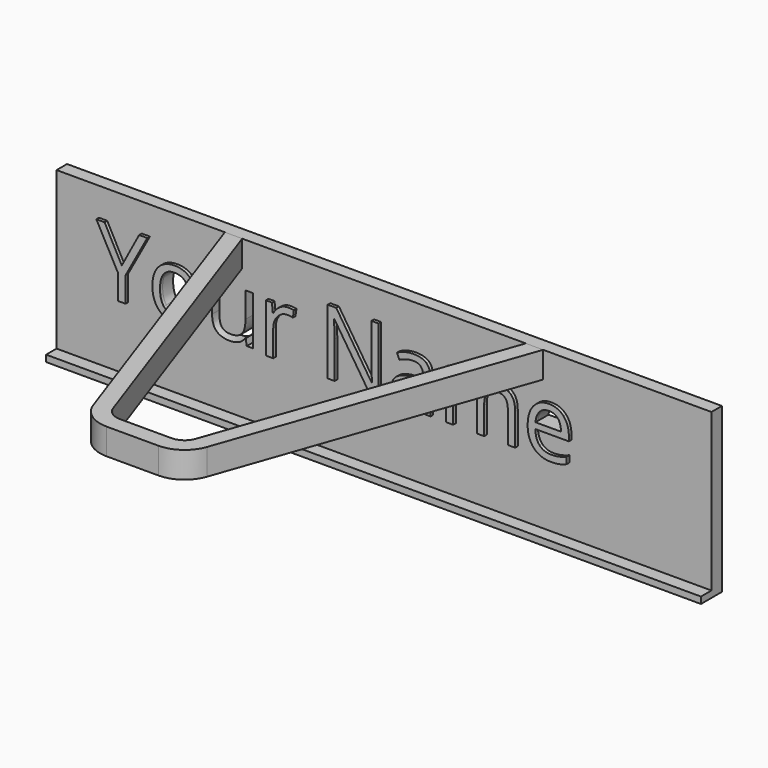
from build123d import *

# Parameters (mm, degrees)
F0_W     = 100
F0_H     = 22
F0_H_2   = 2
F1_DEPTH = 2
F0_H_3   = 1
F2_DEPTH = 4
F4_DEPTH = 4
F5_DEPTH = 2.5


# Not quite as in the source:
# - a feature names something its author has since deleted; it is built from what else it names


with BuildPart() as f1:
    # F0 (on Front) → F1 (new body)
    with BuildSketch(Plane.XZ):
        with Locations((-50, 12)):
            Rectangle(F0_W, F0_H)
        with BuildLine():
            add(Edge.make_bspline(
                [(-79.0596093072, 17.3149081237), (-78.1405554877, 16.2764966653), (-78.1405554877, 14.5078334709)],
                knots=[0, 0, 0, 1, 1, 1], degree=2))
            add(Edge.make_bspline(
                [(-78.1405554877, 14.5078334709), (-78.1405554877, 12.689257082), (-79.0552690294, 11.6682067348)],
                knots=[0, 0, 0, 1, 1, 1], degree=2))
            add(Edge.make_bspline(
                [(-79.0552690294, 11.6682067348), (-79.9699825711, 10.6471563876), (-81.5845659044, 10.6471563876)],
                knots=[0, 0, 0, 1, 1, 1], degree=2))
            add(Edge.make_bspline(
                [(-81.5845659044, 10.6471563876), (-82.5828297933, 10.6471563876), (-83.3553992377, 11.1159063876)],
                knots=[0, 0, 0, 1, 1, 1], degree=2))
            add(Edge.make_bspline(
                [(-83.3553992377, 11.1159063876), (-84.1279686822, 11.5846563876), (-84.5489756266, 12.4592223598)],
                knots=[0, 0, 0, 1, 1, 1], degree=2))
            add(Edge.make_bspline(
                [(-84.5489756266, 12.4592223598), (-84.9699825711, 13.333788332), (-84.9699825711, 14.5078334709)],
                knots=[0, 0, 0, 1, 1, 1], degree=2))
            add(Edge.make_bspline(
                [(-84.9699825711, 14.5078334709), (-84.9699825711, 16.3242397209), (-84.0606943766, 17.3387796515)],
                knots=[0, 0, 0, 1, 1, 1], degree=2))
            add(Edge.make_bspline(
                [(-84.0606943766, 17.3387796515), (-83.1514061822, 18.353319582), (-81.5368228488, 18.353319582)],
                knots=[0, 0, 0, 1, 1, 1], degree=2))
            add(Edge.make_bspline(
                [(-81.5368228488, 18.353319582), (-79.9786631266, 18.353319582), (-79.0596093072, 17.3149081237)],
                knots=[0, 0, 0, 1, 1, 1], degree=2))
        make_face(mode=Mode.SUBTRACT)
        Polygon((-92.2659895155, 20.6992397209), (-89.64012146, 15.7404723598), (-86.9968922933, 20.6992397209), (-85.7490624322, 20.6992397209), (-89.0585242377, 14.6293612487), (-89.0585242377, 10.7838751376), (-90.2238888211, 10.7838751376), (-90.2238888211, 14.5751077765), (-93.52684021, 20.6992397209), align=None, mode=Mode.SUBTRACT)
        with BuildLine():
            Line((-76.2460242377, 18.216600832), (-75.1067013211, 18.216600832))
            Line((-75.1067013211, 18.216600832), (-75.1067013211, 13.3945522209))
            add(Edge.make_bspline(
                [(-75.1067013211, 13.3945522209), (-75.1067013211, 12.4852640265), (-74.6932898627, 12.0382154153)],
                knots=[0, 0, 0, 1, 1, 1], degree=2))
            add(Edge.make_bspline(
                [(-74.6932898627, 12.0382154153), (-74.2798784044, 11.5911668042), (-73.3988020155, 11.5911668042)],
                knots=[0, 0, 0, 1, 1, 1], degree=2))
            add(Edge.make_bspline(
                [(-73.3988020155, 11.5911668042), (-72.2312672933, 11.5911668042), (-71.6930728488, 12.2281025681)],
                knots=[0, 0, 0, 1, 1, 1], degree=2))
            add(Edge.make_bspline(
                [(-71.6930728488, 12.2281025681), (-71.1548784044, 12.865038332), (-71.1548784044, 14.310350832)],
                knots=[0, 0, 0, 1, 1, 1], degree=2))
            Line((-71.1548784044, 14.310350832), (-71.1548784044, 18.216600832))
            Line((-71.1548784044, 18.216600832), (-70.0285763211, 18.216600832))
            Line((-70.0285763211, 18.216600832), (-70.0285763211, 10.7838751376))
            Line((-70.0285763211, 10.7838751376), (-70.9573957655, 10.7838751376))
            Line((-70.9573957655, 10.7838751376), (-71.1201561822, 11.7799688876))
            Line((-71.1201561822, 11.7799688876), (-71.1809200711, 11.7799688876))
            add(Edge.make_bspline(
                [(-71.1809200711, 11.7799688876), (-71.5259721544, 11.2309237487), (-72.14012146, 10.9390400681)],
                knots=[0, 0, 0, 1, 1, 1], degree=2))
            add(Edge.make_bspline(
                [(-72.14012146, 10.9390400681), (-72.7542707655, 10.6471563876), (-73.5420311822, 10.6471563876)],
                knots=[0, 0, 0, 1, 1, 1], degree=2))
            add(Edge.make_bspline(
                [(-73.5420311822, 10.6471563876), (-74.8983679877, 10.6471563876), (-75.5721961127, 11.2916876376)],
                knots=[0, 0, 0, 1, 1, 1], degree=2))
            add(Edge.make_bspline(
                [(-75.5721961127, 11.2916876376), (-76.2460242377, 11.9362188876), (-76.2460242377, 13.353319582)],
                knots=[0, 0, 0, 1, 1, 1], degree=2))
            Line((-76.2460242377, 13.353319582), (-76.2460242377, 18.216600832))
        make_face(mode=Mode.SUBTRACT)
        with BuildLine():
            add(Edge.make_bspline(
                [(-65.5320485433, 17.9594393737), (-64.9482811822, 18.353319582), (-64.24949646, 18.353319582)],
                knots=[0, 0, 0, 1, 1, 1], degree=2))
            add(Edge.make_bspline(
                [(-64.24949646, 18.353319582), (-63.7547047933, 18.353319582), (-63.3619096544, 18.2708543042)],
                knots=[0, 0, 0, 1, 1, 1], degree=2))
            Line((-63.3619096544, 18.2708543042), (-63.5181596544, 17.2270174987))
            add(Edge.make_bspline(
                [(-63.5181596544, 17.2270174987), (-63.9782290988, 17.3290140265), (-64.3319617377, 17.3290140265)],
                knots=[0, 0, 0, 1, 1, 1], degree=2))
            add(Edge.make_bspline(
                [(-64.3319617377, 17.3290140265), (-65.2347395155, 17.3290140265), (-65.8749304877, 16.5965921515)],
                knots=[0, 0, 0, 1, 1, 1], degree=2))
            add(Edge.make_bspline(
                [(-65.8749304877, 16.5965921515), (-66.51512146, 15.8641702765), (-66.51512146, 14.7725904153)],
                knots=[0, 0, 0, 1, 1, 1], degree=2))
            Line((-66.51512146, 14.7725904153), (-66.51512146, 10.7838751376))
            Line((-66.51512146, 10.7838751376), (-67.6414235433, 10.7838751376))
            Line((-67.6414235433, 10.7838751376), (-67.6414235433, 18.216600832))
            Line((-67.6414235433, 18.216600832), (-66.7126040988, 18.216600832))
            Line((-66.7126040988, 18.216600832), (-66.5823957655, 16.8407327765))
            Line((-66.5823957655, 16.8407327765), (-66.5281422933, 16.8407327765))
            add(Edge.make_bspline(
                [(-66.5281422933, 16.8407327765), (-66.1158159044, 17.5655591653), (-65.5320485433, 17.9594393737)],
                knots=[0, 0, 0, 1, 1, 1], degree=2))
        make_face(mode=Mode.SUBTRACT)
        with BuildLine():
            Line((-50.4474131266, 20.6992397209), (-50.4474131266, 10.7838751376))
            Line((-50.4474131266, 10.7838751376), (-51.7625172933, 10.7838751376))
            Line((-51.7625172933, 10.7838751376), (-57.1813540988, 19.1041876376))
            Line((-57.1813540988, 19.1041876376), (-57.2356075711, 19.1041876376))
            add(Edge.make_bspline(
                [(-57.2356075711, 19.1041876376), (-57.1271006266, 17.6393438876), (-57.1271006266, 16.419725832)],
                knots=[0, 0, 0, 1, 1, 1], degree=2))
            Line((-57.1271006266, 16.419725832), (-57.1271006266, 10.7838751376))
            Line((-57.1271006266, 10.7838751376), (-58.1926388211, 10.7838751376))
            Line((-58.1926388211, 10.7838751376), (-58.1926388211, 20.6992397209))
            Line((-58.1926388211, 20.6992397209), (-56.8905554877, 20.6992397209))
            Line((-56.8905554877, 20.6992397209), (-51.4847395155, 12.4114793042))
            Line((-51.4847395155, 12.4114793042), (-51.4304860433, 12.4114793042))
            add(Edge.make_bspline(
                [(-51.4304860433, 12.4114793042), (-51.4435068766, 12.5937709709), (-51.4912499322, 13.587694582)],
                knots=[0, 0, 0, 1, 1, 1], degree=2))
            add(Edge.make_bspline(
                [(-51.4912499322, 13.587694582), (-51.5389929877, 14.5816181931), (-51.5259721544, 15.0091355542)],
                knots=[0, 0, 0, 1, 1, 1], degree=2))
            Line((-51.5259721544, 15.0091355542), (-51.5259721544, 20.6992397209))
            Line((-51.5259721544, 20.6992397209), (-50.4474131266, 20.6992397209))
        make_face(mode=Mode.SUBTRACT)
        with BuildLine():
            Line((-42.4851735433, 10.7838751376), (-43.3206770155, 10.7838751376))
            Line((-43.3206770155, 10.7838751376), (-43.5442013211, 11.8429029153))
            Line((-43.5442013211, 11.8429029153), (-43.5984547933, 11.8429029153))
            add(Edge.make_bspline(
                [(-43.5984547933, 11.8429029153), (-44.1540103488, 11.1441181931), (-44.7063106961, 10.8956372903)],
                knots=[0, 0, 0, 1, 1, 1], degree=2))
            add(Edge.make_bspline(
                [(-44.7063106961, 10.8956372903), (-45.2586110433, 10.6471563876), (-46.0876040988, 10.6471563876)],
                knots=[0, 0, 0, 1, 1, 1], degree=2))
            add(Edge.make_bspline(
                [(-46.0876040988, 10.6471563876), (-47.1922047933, 10.6471563876), (-47.8193749322, 11.2179029153)],
                knots=[0, 0, 0, 1, 1, 1], degree=2))
            add(Edge.make_bspline(
                [(-47.8193749322, 11.2179029153), (-48.4465450711, 11.7886494431), (-48.4465450711, 12.8389966653)],
                knots=[0, 0, 0, 1, 1, 1], degree=2))
            add(Edge.make_bspline(
                [(-48.4465450711, 12.8389966653), (-48.4465450711, 15.0894306931), (-44.8462846544, 15.1979376376)],
                knots=[0, 0, 0, 1, 1, 1], degree=2))
            Line((-44.8462846544, 15.1979376376), (-43.58543396, 15.2391702765))
            Line((-43.58543396, 15.2391702765), (-43.58543396, 15.7014098598))
            add(Edge.make_bspline(
                [(-43.58543396, 15.7014098598), (-43.58543396, 16.575975832), (-43.9608679877, 16.9926424987)],
                knots=[0, 0, 0, 1, 1, 1], degree=2))
            add(Edge.make_bspline(
                [(-43.9608679877, 16.9926424987), (-44.3363020155, 17.4093091653), (-45.1652950711, 17.4093091653)],
                knots=[0, 0, 0, 1, 1, 1], degree=2))
            add(Edge.make_bspline(
                [(-45.1652950711, 17.4093091653), (-46.0941145155, 17.4093091653), (-47.2659895155, 16.8407327765)],
                knots=[0, 0, 0, 1, 1, 1], degree=2))
            Line((-47.2659895155, 16.8407327765), (-47.6132117377, 17.7022779153))
            add(Edge.make_bspline(
                [(-47.6132117377, 17.7022779153), (-47.0641665988, 17.9995869431), (-46.4098697238, 18.1688577765)],
                knots=[0, 0, 0, 1, 1, 1], degree=2))
            add(Edge.make_bspline(
                [(-46.4098697238, 18.1688577765), (-45.7555728488, 18.3381286098), (-45.0958506266, 18.3381286098)],
                knots=[0, 0, 0, 1, 1, 1], degree=2))
            add(Edge.make_bspline(
                [(-45.0958506266, 18.3381286098), (-43.7677256266, 18.3381286098), (-43.126449585, 17.7489359015)],
                knots=[0, 0, 0, 1, 1, 1], degree=2))
            add(Edge.make_bspline(
                [(-43.126449585, 17.7489359015), (-42.4851735433, 17.1597431931), (-42.4851735433, 15.8576598598)],
                knots=[0, 0, 0, 1, 1, 1], degree=2))
            Line((-42.4851735433, 15.8576598598), (-42.4851735433, 10.7838751376))
        make_face(mode=Mode.SUBTRACT)
        with BuildLine():
            Line((-29.5685068766, 10.7838751376), (-30.6926388211, 10.7838751376))
            Line((-30.6926388211, 10.7838751376), (-30.6926388211, 15.618944582))
            add(Edge.make_bspline(
                [(-30.6926388211, 15.618944582), (-30.6926388211, 16.5087015265), (-31.0724131266, 16.9524949292)],
                knots=[0, 0, 0, 1, 1, 1], degree=2))
            add(Edge.make_bspline(
                [(-31.0724131266, 16.9524949292), (-31.4521874322, 17.396288332), (-32.2529686822, 17.396288332)],
                knots=[0, 0, 0, 1, 1, 1], degree=2))
            add(Edge.make_bspline(
                [(-32.2529686822, 17.396288332), (-33.3033159044, 17.396288332), (-33.8057030572, 16.7929897209)],
                knots=[0, 0, 0, 1, 1, 1], degree=2))
            add(Edge.make_bspline(
                [(-33.8057030572, 16.7929897209), (-34.30809021, 16.1896911098), (-34.30809021, 14.935350832)],
                knots=[0, 0, 0, 1, 1, 1], degree=2))
            Line((-34.30809021, 14.935350832), (-34.30809021, 10.7838751376))
            Line((-34.30809021, 10.7838751376), (-35.4343922933, 10.7838751376))
            Line((-35.4343922933, 10.7838751376), (-35.4343922933, 15.618944582))
            add(Edge.make_bspline(
                [(-35.4343922933, 15.618944582), (-35.4343922933, 16.5087015265), (-35.8141665988, 16.9524949292)],
                knots=[0, 0, 0, 1, 1, 1], degree=2))
            add(Edge.make_bspline(
                [(-35.8141665988, 16.9524949292), (-36.1939409044, 17.396288332), (-37.0012325711, 17.396288332)],
                knots=[0, 0, 0, 1, 1, 1], degree=2))
            add(Edge.make_bspline(
                [(-37.0012325711, 17.396288332), (-38.05809021, 17.396288332), (-38.5496266683, 16.7626077765)],
                knots=[0, 0, 0, 1, 1, 1], degree=2))
            add(Edge.make_bspline(
                [(-38.5496266683, 16.7626077765), (-39.0411631266, 16.1289272209), (-39.0411631266, 14.6836147209)],
                knots=[0, 0, 0, 1, 1, 1], degree=2))
            Line((-39.0411631266, 14.6836147209), (-39.0411631266, 10.7838751376))
            Line((-39.0411631266, 10.7838751376), (-40.16746521, 10.7838751376))
            Line((-40.16746521, 10.7838751376), (-40.16746521, 18.216600832))
            Line((-40.16746521, 18.216600832), (-39.2516665988, 18.216600832))
            Line((-39.2516665988, 18.216600832), (-39.0693749322, 17.1988056931))
            Line((-39.0693749322, 17.1988056931), (-39.01512146, 17.1988056931))
            add(Edge.make_bspline(
                [(-39.01512146, 17.1988056931), (-38.6961110433, 17.7413404153), (-38.1155988905, 18.0473299987)],
                knots=[0, 0, 0, 1, 1, 1], degree=2))
            add(Edge.make_bspline(
                [(-38.1155988905, 18.0473299987), (-37.5350867377, 18.353319582), (-36.8167707655, 18.353319582)],
                knots=[0, 0, 0, 1, 1, 1], degree=2))
            add(Edge.make_bspline(
                [(-36.8167707655, 18.353319582), (-35.0741492377, 18.353319582), (-34.5381249322, 17.0902987487)],
                knots=[0, 0, 0, 1, 1, 1], degree=2))
            Line((-34.5381249322, 17.0902987487), (-34.48387146, 17.0902987487))
            add(Edge.make_bspline(
                [(-34.48387146, 17.0902987487), (-34.15184021, 17.6740661098), (-33.5214148627, 18.0136928459)],
                knots=[0, 0, 0, 1, 1, 1], degree=2))
            add(Edge.make_bspline(
                [(-33.5214148627, 18.0136928459), (-32.8909895155, 18.353319582), (-32.0836978488, 18.353319582)],
                knots=[0, 0, 0, 1, 1, 1], degree=2))
            add(Edge.make_bspline(
                [(-32.0836978488, 18.353319582), (-30.8228471544, 18.353319582), (-30.1956770155, 17.7055331237)],
                knots=[0, 0, 0, 1, 1, 1], degree=2))
            add(Edge.make_bspline(
                [(-30.1956770155, 17.7055331237), (-29.5685068766, 17.0577466653), (-29.5685068766, 15.6319654153)],
                knots=[0, 0, 0, 1, 1, 1], degree=2))
            Line((-29.5685068766, 15.6319654153), (-29.5685068766, 10.7838751376))
        make_face(mode=Mode.SUBTRACT)
        with BuildLine():
            add(Edge.make_bspline(
                [(-22.82371521, 10.7600036098), (-23.3553992377, 10.6471563876), (-24.1084374322, 10.6471563876)],
                knots=[0, 0, 0, 1, 1, 1], degree=2))
            add(Edge.make_bspline(
                [(-24.1084374322, 10.6471563876), (-25.7555728488, 10.6471563876), (-26.7093488905, 11.6519306931)],
                knots=[0, 0, 0, 1, 1, 1], degree=2))
            add(Edge.make_bspline(
                [(-26.7093488905, 11.6519306931), (-27.6631249322, 12.6567049987), (-27.6631249322, 14.4383890265)],
                knots=[0, 0, 0, 1, 1, 1], degree=2))
            add(Edge.make_bspline(
                [(-27.6631249322, 14.4383890265), (-27.6631249322, 16.2374341653), (-26.7777082655, 17.2953768737)],
                knots=[0, 0, 0, 1, 1, 1], degree=2))
            add(Edge.make_bspline(
                [(-26.7777082655, 17.2953768737), (-25.8922915988, 18.353319582), (-24.3992360433, 18.353319582)],
                knots=[0, 0, 0, 1, 1, 1], degree=2))
            add(Edge.make_bspline(
                [(-24.3992360433, 18.353319582), (-23.0038367377, 18.353319582), (-22.1900346544, 17.4342657626)],
                knots=[0, 0, 0, 1, 1, 1], degree=2))
            add(Edge.make_bspline(
                [(-22.1900346544, 17.4342657626), (-21.3762325711, 16.5152119431), (-21.3762325711, 15.0091355542)],
                knots=[0, 0, 0, 1, 1, 1], degree=2))
            Line((-21.3762325711, 15.0091355542), (-21.3762325711, 14.2973299987))
            Line((-21.3762325711, 14.2973299987), (-26.49559021, 14.2973299987))
            add(Edge.make_bspline(
                [(-26.49559021, 14.2973299987), (-26.4608679877, 12.9887362487), (-25.8336978488, 12.3105678459)],
                knots=[0, 0, 0, 1, 1, 1], degree=2))
            add(Edge.make_bspline(
                [(-25.8336978488, 12.3105678459), (-25.20652771, 11.6323994431), (-24.0672047933, 11.6323994431)],
                knots=[0, 0, 0, 1, 1, 1], degree=2))
            add(Edge.make_bspline(
                [(-24.0672047933, 11.6323994431), (-22.8671179877, 11.6323994431), (-21.6952429877, 12.1337015265)],
                knots=[0, 0, 0, 1, 1, 1], degree=2))
            Line((-21.6952429877, 12.1337015265), (-21.6952429877, 11.1289272209))
            add(Edge.make_bspline(
                [(-21.6952429877, 11.1289272209), (-22.2920311822, 10.872850832), (-22.82371521, 10.7600036098)],
                knots=[0, 0, 0, 1, 1, 1], degree=2))
        make_face(mode=Mode.SUBTRACT)
        with Locations((-50, 24)):
            Rectangle(F0_W, F0_H_2)
        with BuildLine():
            add(Edge.make_bspline(
                [(-78.1405554877, 14.5078334709), (-78.1405554877, 12.689257082), (-79.0552690294, 11.6682067348)],
                knots=[0, 0, 0, 1, 1, 1], degree=2))
            add(Edge.make_bspline(
                [(-79.0596093072, 17.3149081237), (-78.1405554877, 16.2764966653), (-78.1405554877, 14.5078334709)],
                knots=[0, 0, 0, 1, 1, 1], degree=2))
            add(Edge.make_bspline(
                [(-81.5368228488, 18.353319582), (-79.9786631266, 18.353319582), (-79.0596093072, 17.3149081237)],
                knots=[0, 0, 0, 1, 1, 1], degree=2))
            add(Edge.make_bspline(
                [(-84.0606943766, 17.3387796515), (-83.1514061822, 18.353319582), (-81.5368228488, 18.353319582)],
                knots=[0, 0, 0, 1, 1, 1], degree=2))
            add(Edge.make_bspline(
                [(-84.9699825711, 14.5078334709), (-84.9699825711, 16.3242397209), (-84.0606943766, 17.3387796515)],
                knots=[0, 0, 0, 1, 1, 1], degree=2))
            add(Edge.make_bspline(
                [(-84.5489756266, 12.4592223598), (-84.9699825711, 13.333788332), (-84.9699825711, 14.5078334709)],
                knots=[0, 0, 0, 1, 1, 1], degree=2))
            add(Edge.make_bspline(
                [(-83.3553992377, 11.1159063876), (-84.1279686822, 11.5846563876), (-84.5489756266, 12.4592223598)],
                knots=[0, 0, 0, 1, 1, 1], degree=2))
            add(Edge.make_bspline(
                [(-81.5845659044, 10.6471563876), (-82.5828297933, 10.6471563876), (-83.3553992377, 11.1159063876)],
                knots=[0, 0, 0, 1, 1, 1], degree=2))
            add(Edge.make_bspline(
                [(-79.0552690294, 11.6682067348), (-79.9699825711, 10.6471563876), (-81.5845659044, 10.6471563876)],
                knots=[0, 0, 0, 1, 1, 1], degree=2))
        make_face()
        with BuildLine():
            add(Edge.make_bspline(
                [(-83.8024478488, 14.5078334709), (-83.8024478488, 13.0820522209), (-83.2327863905, 12.3366095126)],
                knots=[0, 0, 0, 1, 1, 1], degree=2))
            add(Edge.make_bspline(
                [(-83.2392968072, 16.6703768737), (-83.8024478488, 15.9444654153), (-83.8024478488, 14.5078334709)],
                knots=[0, 0, 0, 1, 1, 1], degree=2))
            add(Edge.make_bspline(
                [(-81.5715450711, 17.396288332), (-82.6761457655, 17.396288332), (-83.2392968072, 16.6703768737)],
                knots=[0, 0, 0, 1, 1, 1], degree=2))
            add(Edge.make_bspline(
                [(-79.8788367377, 16.6606112487), (-80.4517534044, 17.396288332), (-81.5715450711, 17.396288332)],
                knots=[0, 0, 0, 1, 1, 1], degree=2))
            add(Edge.make_bspline(
                [(-79.3059200711, 14.5078334709), (-79.3059200711, 15.9249341653), (-79.8788367377, 16.6606112487)],
                knots=[0, 0, 0, 1, 1, 1], degree=2))
            add(Edge.make_bspline(
                [(-79.8788367377, 12.3333543042), (-79.3059200711, 13.0755418042), (-79.3059200711, 14.5078334709)],
                knots=[0, 0, 0, 1, 1, 1], degree=2))
            add(Edge.make_bspline(
                [(-81.5585242377, 11.5911668042), (-80.4517534044, 11.5911668042), (-79.8788367377, 12.3333543042)],
                knots=[0, 0, 0, 1, 1, 1], degree=2))
            add(Edge.make_bspline(
                [(-83.2327863905, 12.3366095126), (-82.6631249322, 11.5911668042), (-81.5585242377, 11.5911668042)],
                knots=[0, 0, 0, 1, 1, 1], degree=2))
        make_face(mode=Mode.SUBTRACT)
        with BuildLine():
            Line((-51.7625172933, 10.7838751376), (-50.4474131266, 10.7838751376))
            Line((-50.4474131266, 10.7838751376), (-50.4474131266, 20.6992397209))
            Line((-50.4474131266, 20.6992397209), (-51.5259721544, 20.6992397209))
            Line((-51.5259721544, 20.6992397209), (-51.5259721544, 15.0091355542))
            add(Edge.make_bspline(
                [(-51.4912499322, 13.587694582), (-51.5389929877, 14.5816181931), (-51.5259721544, 15.0091355542)],
                knots=[0, 0, 0, 1, 1, 1], degree=2))
            add(Edge.make_bspline(
                [(-51.4304860433, 12.4114793042), (-51.4435068766, 12.5937709709), (-51.4912499322, 13.587694582)],
                knots=[0, 0, 0, 1, 1, 1], degree=2))
            Line((-51.4304860433, 12.4114793042), (-51.4847395155, 12.4114793042))
            Line((-51.4847395155, 12.4114793042), (-56.8905554877, 20.6992397209))
            Line((-56.8905554877, 20.6992397209), (-58.1926388211, 20.6992397209))
            Line((-58.1926388211, 20.6992397209), (-58.1926388211, 10.7838751376))
            Line((-58.1926388211, 10.7838751376), (-57.1271006266, 10.7838751376))
            Line((-57.1271006266, 10.7838751376), (-57.1271006266, 16.419725832))
            add(Edge.make_bspline(
                [(-57.2356075711, 19.1041876376), (-57.1271006266, 17.6393438876), (-57.1271006266, 16.419725832)],
                knots=[0, 0, 0, 1, 1, 1], degree=2))
            Line((-57.2356075711, 19.1041876376), (-57.1813540988, 19.1041876376))
            Line((-57.1813540988, 19.1041876376), (-51.7625172933, 10.7838751376))
        make_face()
        with BuildLine():
            Line((-30.6926388211, 15.618944582), (-30.6926388211, 10.7838751376))
            Line((-30.6926388211, 10.7838751376), (-29.5685068766, 10.7838751376))
            Line((-29.5685068766, 10.7838751376), (-29.5685068766, 15.6319654153))
            add(Edge.make_bspline(
                [(-30.1956770155, 17.7055331237), (-29.5685068766, 17.0577466653), (-29.5685068766, 15.6319654153)],
                knots=[0, 0, 0, 1, 1, 1], degree=2))
            add(Edge.make_bspline(
                [(-32.0836978488, 18.353319582), (-30.8228471544, 18.353319582), (-30.1956770155, 17.7055331237)],
                knots=[0, 0, 0, 1, 1, 1], degree=2))
            add(Edge.make_bspline(
                [(-33.5214148627, 18.0136928459), (-32.8909895155, 18.353319582), (-32.0836978488, 18.353319582)],
                knots=[0, 0, 0, 1, 1, 1], degree=2))
            add(Edge.make_bspline(
                [(-34.48387146, 17.0902987487), (-34.15184021, 17.6740661098), (-33.5214148627, 18.0136928459)],
                knots=[0, 0, 0, 1, 1, 1], degree=2))
            Line((-34.48387146, 17.0902987487), (-34.5381249322, 17.0902987487))
            add(Edge.make_bspline(
                [(-36.8167707655, 18.353319582), (-35.0741492377, 18.353319582), (-34.5381249322, 17.0902987487)],
                knots=[0, 0, 0, 1, 1, 1], degree=2))
            add(Edge.make_bspline(
                [(-38.1155988905, 18.0473299987), (-37.5350867377, 18.353319582), (-36.8167707655, 18.353319582)],
                knots=[0, 0, 0, 1, 1, 1], degree=2))
            add(Edge.make_bspline(
                [(-39.01512146, 17.1988056931), (-38.6961110433, 17.7413404153), (-38.1155988905, 18.0473299987)],
                knots=[0, 0, 0, 1, 1, 1], degree=2))
            Line((-39.01512146, 17.1988056931), (-39.0693749322, 17.1988056931))
            Line((-39.0693749322, 17.1988056931), (-39.2516665988, 18.216600832))
            Line((-39.2516665988, 18.216600832), (-40.16746521, 18.216600832))
            Line((-40.16746521, 18.216600832), (-40.16746521, 10.7838751376))
            Line((-40.16746521, 10.7838751376), (-39.0411631266, 10.7838751376))
            Line((-39.0411631266, 10.7838751376), (-39.0411631266, 14.6836147209))
            add(Edge.make_bspline(
                [(-38.5496266683, 16.7626077765), (-39.0411631266, 16.1289272209), (-39.0411631266, 14.6836147209)],
                knots=[0, 0, 0, 1, 1, 1], degree=2))
            add(Edge.make_bspline(
                [(-37.0012325711, 17.396288332), (-38.05809021, 17.396288332), (-38.5496266683, 16.7626077765)],
                knots=[0, 0, 0, 1, 1, 1], degree=2))
            add(Edge.make_bspline(
                [(-35.8141665988, 16.9524949292), (-36.1939409044, 17.396288332), (-37.0012325711, 17.396288332)],
                knots=[0, 0, 0, 1, 1, 1], degree=2))
            add(Edge.make_bspline(
                [(-35.4343922933, 15.618944582), (-35.4343922933, 16.5087015265), (-35.8141665988, 16.9524949292)],
                knots=[0, 0, 0, 1, 1, 1], degree=2))
            Line((-35.4343922933, 15.618944582), (-35.4343922933, 10.7838751376))
            Line((-35.4343922933, 10.7838751376), (-34.30809021, 10.7838751376))
            Line((-34.30809021, 10.7838751376), (-34.30809021, 14.935350832))
            add(Edge.make_bspline(
                [(-33.8057030572, 16.7929897209), (-34.30809021, 16.1896911098), (-34.30809021, 14.935350832)],
                knots=[0, 0, 0, 1, 1, 1], degree=2))
            add(Edge.make_bspline(
                [(-32.2529686822, 17.396288332), (-33.3033159044, 17.396288332), (-33.8057030572, 16.7929897209)],
                knots=[0, 0, 0, 1, 1, 1], degree=2))
            add(Edge.make_bspline(
                [(-31.0724131266, 16.9524949292), (-31.4521874322, 17.396288332), (-32.2529686822, 17.396288332)],
                knots=[0, 0, 0, 1, 1, 1], degree=2))
            add(Edge.make_bspline(
                [(-30.6926388211, 15.618944582), (-30.6926388211, 16.5087015265), (-31.0724131266, 16.9524949292)],
                knots=[0, 0, 0, 1, 1, 1], degree=2))
        make_face()
        with BuildLine():
            Line((-43.5442013211, 11.8429029153), (-43.3206770155, 10.7838751376))
            Line((-43.3206770155, 10.7838751376), (-42.4851735433, 10.7838751376))
            Line((-42.4851735433, 10.7838751376), (-42.4851735433, 15.8576598598))
            add(Edge.make_bspline(
                [(-43.126449585, 17.7489359015), (-42.4851735433, 17.1597431931), (-42.4851735433, 15.8576598598)],
                knots=[0, 0, 0, 1, 1, 1], degree=2))
            add(Edge.make_bspline(
                [(-45.0958506266, 18.3381286098), (-43.7677256266, 18.3381286098), (-43.126449585, 17.7489359015)],
                knots=[0, 0, 0, 1, 1, 1], degree=2))
            add(Edge.make_bspline(
                [(-46.4098697238, 18.1688577765), (-45.7555728488, 18.3381286098), (-45.0958506266, 18.3381286098)],
                knots=[0, 0, 0, 1, 1, 1], degree=2))
            add(Edge.make_bspline(
                [(-47.6132117377, 17.7022779153), (-47.0641665988, 17.9995869431), (-46.4098697238, 18.1688577765)],
                knots=[0, 0, 0, 1, 1, 1], degree=2))
            Line((-47.6132117377, 17.7022779153), (-47.2659895155, 16.8407327765))
            add(Edge.make_bspline(
                [(-45.1652950711, 17.4093091653), (-46.0941145155, 17.4093091653), (-47.2659895155, 16.8407327765)],
                knots=[0, 0, 0, 1, 1, 1], degree=2))
            add(Edge.make_bspline(
                [(-43.9608679877, 16.9926424987), (-44.3363020155, 17.4093091653), (-45.1652950711, 17.4093091653)],
                knots=[0, 0, 0, 1, 1, 1], degree=2))
            add(Edge.make_bspline(
                [(-43.58543396, 15.7014098598), (-43.58543396, 16.575975832), (-43.9608679877, 16.9926424987)],
                knots=[0, 0, 0, 1, 1, 1], degree=2))
            Line((-43.58543396, 15.7014098598), (-43.58543396, 15.2391702765))
            Line((-43.58543396, 15.2391702765), (-44.8462846544, 15.1979376376))
            add(Edge.make_bspline(
                [(-48.4465450711, 12.8389966653), (-48.4465450711, 15.0894306931), (-44.8462846544, 15.1979376376)],
                knots=[0, 0, 0, 1, 1, 1], degree=2))
            add(Edge.make_bspline(
                [(-47.8193749322, 11.2179029153), (-48.4465450711, 11.7886494431), (-48.4465450711, 12.8389966653)],
                knots=[0, 0, 0, 1, 1, 1], degree=2))
            add(Edge.make_bspline(
                [(-46.0876040988, 10.6471563876), (-47.1922047933, 10.6471563876), (-47.8193749322, 11.2179029153)],
                knots=[0, 0, 0, 1, 1, 1], degree=2))
            add(Edge.make_bspline(
                [(-44.7063106961, 10.8956372903), (-45.2586110433, 10.6471563876), (-46.0876040988, 10.6471563876)],
                knots=[0, 0, 0, 1, 1, 1], degree=2))
            add(Edge.make_bspline(
                [(-43.5984547933, 11.8429029153), (-44.1540103488, 11.1441181931), (-44.7063106961, 10.8956372903)],
                knots=[0, 0, 0, 1, 1, 1], degree=2))
            Line((-43.5984547933, 11.8429029153), (-43.5442013211, 11.8429029153))
        make_face()
        with BuildLine():
            add(Edge.make_bspline(
                [(-45.8640797933, 11.5781459709), (-44.8115624322, 11.5781459709), (-44.2115190294, 12.1543178459)],
                knots=[0, 0, 0, 1, 1, 1], degree=2))
            add(Edge.make_bspline(
                [(-46.8970659044, 11.8960713181), (-46.5281422933, 11.5781459709), (-45.8640797933, 11.5781459709)],
                knots=[0, 0, 0, 1, 1, 1], degree=2))
            add(Edge.make_bspline(
                [(-47.2659895155, 12.825975832), (-47.2659895155, 12.2139966653), (-46.8970659044, 11.8960713181)],
                knots=[0, 0, 0, 1, 1, 1], degree=2))
            add(Edge.make_bspline(
                [(-46.6735415988, 13.9750643737), (-47.2659895155, 13.6050556931), (-47.2659895155, 12.825975832)],
                knots=[0, 0, 0, 1, 1, 1], degree=2))
            add(Edge.make_bspline(
                [(-44.73777771, 14.3928161098), (-46.0810936822, 14.3450730542), (-46.6735415988, 13.9750643737)],
                knots=[0, 0, 0, 1, 1, 1], degree=2))
            Line((-44.73777771, 14.3928161098), (-43.6114756266, 14.4383890265))
            Line((-43.6114756266, 14.4383890265), (-43.6114756266, 13.7678161098))
            add(Edge.make_bspline(
                [(-44.2115190294, 12.1543178459), (-43.6114756266, 12.7304897209), (-43.6114756266, 13.7678161098)],
                knots=[0, 0, 0, 1, 1, 1], degree=2))
        make_face(mode=Mode.SUBTRACT)
        with BuildLine():
            add(Edge.make_bspline(
                [(-24.1084374322, 10.6471563876), (-25.7555728488, 10.6471563876), (-26.7093488905, 11.6519306931)],
                knots=[0, 0, 0, 1, 1, 1], degree=2))
            add(Edge.make_bspline(
                [(-22.82371521, 10.7600036098), (-23.3553992377, 10.6471563876), (-24.1084374322, 10.6471563876)],
                knots=[0, 0, 0, 1, 1, 1], degree=2))
            add(Edge.make_bspline(
                [(-21.6952429877, 11.1289272209), (-22.2920311822, 10.872850832), (-22.82371521, 10.7600036098)],
                knots=[0, 0, 0, 1, 1, 1], degree=2))
            Line((-21.6952429877, 11.1289272209), (-21.6952429877, 12.1337015265))
            add(Edge.make_bspline(
                [(-24.0672047933, 11.6323994431), (-22.8671179877, 11.6323994431), (-21.6952429877, 12.1337015265)],
                knots=[0, 0, 0, 1, 1, 1], degree=2))
            add(Edge.make_bspline(
                [(-25.8336978488, 12.3105678459), (-25.20652771, 11.6323994431), (-24.0672047933, 11.6323994431)],
                knots=[0, 0, 0, 1, 1, 1], degree=2))
            add(Edge.make_bspline(
                [(-26.49559021, 14.2973299987), (-26.4608679877, 12.9887362487), (-25.8336978488, 12.3105678459)],
                knots=[0, 0, 0, 1, 1, 1], degree=2))
            Line((-26.49559021, 14.2973299987), (-21.3762325711, 14.2973299987))
            Line((-21.3762325711, 14.2973299987), (-21.3762325711, 15.0091355542))
            add(Edge.make_bspline(
                [(-22.1900346544, 17.4342657626), (-21.3762325711, 16.5152119431), (-21.3762325711, 15.0091355542)],
                knots=[0, 0, 0, 1, 1, 1], degree=2))
            add(Edge.make_bspline(
                [(-24.3992360433, 18.353319582), (-23.0038367377, 18.353319582), (-22.1900346544, 17.4342657626)],
                knots=[0, 0, 0, 1, 1, 1], degree=2))
            add(Edge.make_bspline(
                [(-26.7777082655, 17.2953768737), (-25.8922915988, 18.353319582), (-24.3992360433, 18.353319582)],
                knots=[0, 0, 0, 1, 1, 1], degree=2))
            add(Edge.make_bspline(
                [(-27.6631249322, 14.4383890265), (-27.6631249322, 16.2374341653), (-26.7777082655, 17.2953768737)],
                knots=[0, 0, 0, 1, 1, 1], degree=2))
            add(Edge.make_bspline(
                [(-26.7093488905, 11.6519306931), (-27.6631249322, 12.6567049987), (-27.6631249322, 14.4383890265)],
                knots=[0, 0, 0, 1, 1, 1], degree=2))
        make_face()
        with BuildLine():
            add(Edge.make_bspline(
                [(-24.4144270155, 17.4093091653), (-25.3085242377, 17.4093091653), (-25.841293335, 16.8266268737)],
                knots=[0, 0, 0, 1, 1, 1], degree=2))
            add(Edge.make_bspline(
                [(-23.0570051405, 16.8429029153), (-23.5311804877, 17.4093091653), (-24.4144270155, 17.4093091653)],
                knots=[0, 0, 0, 1, 1, 1], degree=2))
            add(Edge.make_bspline(
                [(-22.5828297933, 15.2131286098), (-22.5828297933, 16.2764966653), (-23.0570051405, 16.8429029153)],
                knots=[0, 0, 0, 1, 1, 1], degree=2))
            Line((-22.5828297933, 15.2131286098), (-26.4695485433, 15.2131286098))
            add(Edge.make_bspline(
                [(-25.841293335, 16.8266268737), (-26.3740624322, 16.243944582), (-26.4695485433, 15.2131286098)],
                knots=[0, 0, 0, 1, 1, 1], degree=2))
        make_face(mode=Mode.SUBTRACT)
        Polygon((-86.9968922933, 20.6992397209), (-89.64012146, 15.7404723598), (-92.2659895155, 20.6992397209), (-93.52684021, 20.6992397209), (-90.2238888211, 14.5751077765), (-90.2238888211, 10.7838751376), (-89.0585242377, 10.7838751376), (-89.0585242377, 14.6293612487), (-85.7490624322, 20.6992397209), align=None)
        with BuildLine():
            add(Edge.make_bspline(
                [(-64.24949646, 18.353319582), (-63.7547047933, 18.353319582), (-63.3619096544, 18.2708543042)],
                knots=[0, 0, 0, 1, 1, 1], degree=2))
            add(Edge.make_bspline(
                [(-65.5320485433, 17.9594393737), (-64.9482811822, 18.353319582), (-64.24949646, 18.353319582)],
                knots=[0, 0, 0, 1, 1, 1], degree=2))
            add(Edge.make_bspline(
                [(-66.5281422933, 16.8407327765), (-66.1158159044, 17.5655591653), (-65.5320485433, 17.9594393737)],
                knots=[0, 0, 0, 1, 1, 1], degree=2))
            Line((-66.5281422933, 16.8407327765), (-66.5823957655, 16.8407327765))
            Line((-66.5823957655, 16.8407327765), (-66.7126040988, 18.216600832))
            Line((-66.7126040988, 18.216600832), (-67.6414235433, 18.216600832))
            Line((-67.6414235433, 18.216600832), (-67.6414235433, 10.7838751376))
            Line((-67.6414235433, 10.7838751376), (-66.51512146, 10.7838751376))
            Line((-66.51512146, 10.7838751376), (-66.51512146, 14.7725904153))
            add(Edge.make_bspline(
                [(-65.8749304877, 16.5965921515), (-66.51512146, 15.8641702765), (-66.51512146, 14.7725904153)],
                knots=[0, 0, 0, 1, 1, 1], degree=2))
            add(Edge.make_bspline(
                [(-64.3319617377, 17.3290140265), (-65.2347395155, 17.3290140265), (-65.8749304877, 16.5965921515)],
                knots=[0, 0, 0, 1, 1, 1], degree=2))
            add(Edge.make_bspline(
                [(-63.5181596544, 17.2270174987), (-63.9782290988, 17.3290140265), (-64.3319617377, 17.3290140265)],
                knots=[0, 0, 0, 1, 1, 1], degree=2))
            Line((-63.5181596544, 17.2270174987), (-63.3619096544, 18.2708543042))
        make_face()
    extrude(amount=F1_DEPTH)

    # F0 (on Front) → F2 (join)
    with BuildSketch(Plane.XZ):
        with Locations((-50, 0.5)):
            Rectangle(F0_W, F0_H_3)
    extrude(amount=F2_DEPTH)

    # F0 (on Front) → F5 (join)
    with BuildSketch(Plane.XZ):
        Polygon((-86.9968922933, 20.6992397209), (-89.64012146, 15.7404723598), (-92.2659895155, 20.6992397209), (-93.52684021, 20.6992397209), (-90.2238888211, 14.5751077765), (-90.2238888211, 10.7838751376), (-89.0585242377, 10.7838751376), (-89.0585242377, 14.6293612487), (-85.7490624322, 20.6992397209), align=None)
        with BuildLine():
            add(Edge.make_bspline(
                [(-78.1405554877, 14.5078334709), (-78.1405554877, 12.689257082), (-79.0552690294, 11.6682067348)],
                knots=[0, 0, 0, 1, 1, 1], degree=2))
            add(Edge.make_bspline(
                [(-79.0596093072, 17.3149081237), (-78.1405554877, 16.2764966653), (-78.1405554877, 14.5078334709)],
                knots=[0, 0, 0, 1, 1, 1], degree=2))
            add(Edge.make_bspline(
                [(-81.5368228488, 18.353319582), (-79.9786631266, 18.353319582), (-79.0596093072, 17.3149081237)],
                knots=[0, 0, 0, 1, 1, 1], degree=2))
            add(Edge.make_bspline(
                [(-84.0606943766, 17.3387796515), (-83.1514061822, 18.353319582), (-81.5368228488, 18.353319582)],
                knots=[0, 0, 0, 1, 1, 1], degree=2))
            add(Edge.make_bspline(
                [(-84.9699825711, 14.5078334709), (-84.9699825711, 16.3242397209), (-84.0606943766, 17.3387796515)],
                knots=[0, 0, 0, 1, 1, 1], degree=2))
            add(Edge.make_bspline(
                [(-84.5489756266, 12.4592223598), (-84.9699825711, 13.333788332), (-84.9699825711, 14.5078334709)],
                knots=[0, 0, 0, 1, 1, 1], degree=2))
            add(Edge.make_bspline(
                [(-83.3553992377, 11.1159063876), (-84.1279686822, 11.5846563876), (-84.5489756266, 12.4592223598)],
                knots=[0, 0, 0, 1, 1, 1], degree=2))
            add(Edge.make_bspline(
                [(-81.5845659044, 10.6471563876), (-82.5828297933, 10.6471563876), (-83.3553992377, 11.1159063876)],
                knots=[0, 0, 0, 1, 1, 1], degree=2))
            add(Edge.make_bspline(
                [(-79.0552690294, 11.6682067348), (-79.9699825711, 10.6471563876), (-81.5845659044, 10.6471563876)],
                knots=[0, 0, 0, 1, 1, 1], degree=2))
        make_face()
        with BuildLine():
            add(Edge.make_bspline(
                [(-83.8024478488, 14.5078334709), (-83.8024478488, 13.0820522209), (-83.2327863905, 12.3366095126)],
                knots=[0, 0, 0, 1, 1, 1], degree=2))
            add(Edge.make_bspline(
                [(-83.2392968072, 16.6703768737), (-83.8024478488, 15.9444654153), (-83.8024478488, 14.5078334709)],
                knots=[0, 0, 0, 1, 1, 1], degree=2))
            add(Edge.make_bspline(
                [(-81.5715450711, 17.396288332), (-82.6761457655, 17.396288332), (-83.2392968072, 16.6703768737)],
                knots=[0, 0, 0, 1, 1, 1], degree=2))
            add(Edge.make_bspline(
                [(-79.8788367377, 16.6606112487), (-80.4517534044, 17.396288332), (-81.5715450711, 17.396288332)],
                knots=[0, 0, 0, 1, 1, 1], degree=2))
            add(Edge.make_bspline(
                [(-79.3059200711, 14.5078334709), (-79.3059200711, 15.9249341653), (-79.8788367377, 16.6606112487)],
                knots=[0, 0, 0, 1, 1, 1], degree=2))
            add(Edge.make_bspline(
                [(-79.8788367377, 12.3333543042), (-79.3059200711, 13.0755418042), (-79.3059200711, 14.5078334709)],
                knots=[0, 0, 0, 1, 1, 1], degree=2))
            add(Edge.make_bspline(
                [(-81.5585242377, 11.5911668042), (-80.4517534044, 11.5911668042), (-79.8788367377, 12.3333543042)],
                knots=[0, 0, 0, 1, 1, 1], degree=2))
            add(Edge.make_bspline(
                [(-83.2327863905, 12.3366095126), (-82.6631249322, 11.5911668042), (-81.5585242377, 11.5911668042)],
                knots=[0, 0, 0, 1, 1, 1], degree=2))
        make_face(mode=Mode.SUBTRACT)
        with BuildLine():
            add(Edge.make_bspline(
                [(-64.24949646, 18.353319582), (-63.7547047933, 18.353319582), (-63.3619096544, 18.2708543042)],
                knots=[0, 0, 0, 1, 1, 1], degree=2))
            add(Edge.make_bspline(
                [(-65.5320485433, 17.9594393737), (-64.9482811822, 18.353319582), (-64.24949646, 18.353319582)],
                knots=[0, 0, 0, 1, 1, 1], degree=2))
            add(Edge.make_bspline(
                [(-66.5281422933, 16.8407327765), (-66.1158159044, 17.5655591653), (-65.5320485433, 17.9594393737)],
                knots=[0, 0, 0, 1, 1, 1], degree=2))
            Line((-66.5281422933, 16.8407327765), (-66.5823957655, 16.8407327765))
            Line((-66.5823957655, 16.8407327765), (-66.7126040988, 18.216600832))
            Line((-66.7126040988, 18.216600832), (-67.6414235433, 18.216600832))
            Line((-67.6414235433, 18.216600832), (-67.6414235433, 10.7838751376))
            Line((-67.6414235433, 10.7838751376), (-66.51512146, 10.7838751376))
            Line((-66.51512146, 10.7838751376), (-66.51512146, 14.7725904153))
            add(Edge.make_bspline(
                [(-65.8749304877, 16.5965921515), (-66.51512146, 15.8641702765), (-66.51512146, 14.7725904153)],
                knots=[0, 0, 0, 1, 1, 1], degree=2))
            add(Edge.make_bspline(
                [(-64.3319617377, 17.3290140265), (-65.2347395155, 17.3290140265), (-65.8749304877, 16.5965921515)],
                knots=[0, 0, 0, 1, 1, 1], degree=2))
            add(Edge.make_bspline(
                [(-63.5181596544, 17.2270174987), (-63.9782290988, 17.3290140265), (-64.3319617377, 17.3290140265)],
                knots=[0, 0, 0, 1, 1, 1], degree=2))
            Line((-63.5181596544, 17.2270174987), (-63.3619096544, 18.2708543042))
        make_face()
        with BuildLine():
            Line((-51.7625172933, 10.7838751376), (-50.4474131266, 10.7838751376))
            Line((-50.4474131266, 10.7838751376), (-50.4474131266, 20.6992397209))
            Line((-50.4474131266, 20.6992397209), (-51.5259721544, 20.6992397209))
            Line((-51.5259721544, 20.6992397209), (-51.5259721544, 15.0091355542))
            add(Edge.make_bspline(
                [(-51.4912499322, 13.587694582), (-51.5389929877, 14.5816181931), (-51.5259721544, 15.0091355542)],
                knots=[0, 0, 0, 1, 1, 1], degree=2))
            add(Edge.make_bspline(
                [(-51.4304860433, 12.4114793042), (-51.4435068766, 12.5937709709), (-51.4912499322, 13.587694582)],
                knots=[0, 0, 0, 1, 1, 1], degree=2))
            Line((-51.4304860433, 12.4114793042), (-51.4847395155, 12.4114793042))
            Line((-51.4847395155, 12.4114793042), (-56.8905554877, 20.6992397209))
            Line((-56.8905554877, 20.6992397209), (-58.1926388211, 20.6992397209))
            Line((-58.1926388211, 20.6992397209), (-58.1926388211, 10.7838751376))
            Line((-58.1926388211, 10.7838751376), (-57.1271006266, 10.7838751376))
            Line((-57.1271006266, 10.7838751376), (-57.1271006266, 16.419725832))
            add(Edge.make_bspline(
                [(-57.2356075711, 19.1041876376), (-57.1271006266, 17.6393438876), (-57.1271006266, 16.419725832)],
                knots=[0, 0, 0, 1, 1, 1], degree=2))
            Line((-57.2356075711, 19.1041876376), (-57.1813540988, 19.1041876376))
            Line((-57.1813540988, 19.1041876376), (-51.7625172933, 10.7838751376))
        make_face()
        with BuildLine():
            Line((-43.5442013211, 11.8429029153), (-43.3206770155, 10.7838751376))
            Line((-43.3206770155, 10.7838751376), (-42.4851735433, 10.7838751376))
            Line((-42.4851735433, 10.7838751376), (-42.4851735433, 15.8576598598))
            add(Edge.make_bspline(
                [(-43.126449585, 17.7489359015), (-42.4851735433, 17.1597431931), (-42.4851735433, 15.8576598598)],
                knots=[0, 0, 0, 1, 1, 1], degree=2))
            add(Edge.make_bspline(
                [(-45.0958506266, 18.3381286098), (-43.7677256266, 18.3381286098), (-43.126449585, 17.7489359015)],
                knots=[0, 0, 0, 1, 1, 1], degree=2))
            add(Edge.make_bspline(
                [(-46.4098697238, 18.1688577765), (-45.7555728488, 18.3381286098), (-45.0958506266, 18.3381286098)],
                knots=[0, 0, 0, 1, 1, 1], degree=2))
            add(Edge.make_bspline(
                [(-47.6132117377, 17.7022779153), (-47.0641665988, 17.9995869431), (-46.4098697238, 18.1688577765)],
                knots=[0, 0, 0, 1, 1, 1], degree=2))
            Line((-47.6132117377, 17.7022779153), (-47.2659895155, 16.8407327765))
            add(Edge.make_bspline(
                [(-45.1652950711, 17.4093091653), (-46.0941145155, 17.4093091653), (-47.2659895155, 16.8407327765)],
                knots=[0, 0, 0, 1, 1, 1], degree=2))
            add(Edge.make_bspline(
                [(-43.9608679877, 16.9926424987), (-44.3363020155, 17.4093091653), (-45.1652950711, 17.4093091653)],
                knots=[0, 0, 0, 1, 1, 1], degree=2))
            add(Edge.make_bspline(
                [(-43.58543396, 15.7014098598), (-43.58543396, 16.575975832), (-43.9608679877, 16.9926424987)],
                knots=[0, 0, 0, 1, 1, 1], degree=2))
            Line((-43.58543396, 15.7014098598), (-43.58543396, 15.2391702765))
            Line((-43.58543396, 15.2391702765), (-44.8462846544, 15.1979376376))
            add(Edge.make_bspline(
                [(-48.4465450711, 12.8389966653), (-48.4465450711, 15.0894306931), (-44.8462846544, 15.1979376376)],
                knots=[0, 0, 0, 1, 1, 1], degree=2))
            add(Edge.make_bspline(
                [(-47.8193749322, 11.2179029153), (-48.4465450711, 11.7886494431), (-48.4465450711, 12.8389966653)],
                knots=[0, 0, 0, 1, 1, 1], degree=2))
            add(Edge.make_bspline(
                [(-46.0876040988, 10.6471563876), (-47.1922047933, 10.6471563876), (-47.8193749322, 11.2179029153)],
                knots=[0, 0, 0, 1, 1, 1], degree=2))
            add(Edge.make_bspline(
                [(-44.7063106961, 10.8956372903), (-45.2586110433, 10.6471563876), (-46.0876040988, 10.6471563876)],
                knots=[0, 0, 0, 1, 1, 1], degree=2))
            add(Edge.make_bspline(
                [(-43.5984547933, 11.8429029153), (-44.1540103488, 11.1441181931), (-44.7063106961, 10.8956372903)],
                knots=[0, 0, 0, 1, 1, 1], degree=2))
            Line((-43.5984547933, 11.8429029153), (-43.5442013211, 11.8429029153))
        make_face()
        with BuildLine():
            add(Edge.make_bspline(
                [(-45.8640797933, 11.5781459709), (-44.8115624322, 11.5781459709), (-44.2115190294, 12.1543178459)],
                knots=[0, 0, 0, 1, 1, 1], degree=2))
            add(Edge.make_bspline(
                [(-46.8970659044, 11.8960713181), (-46.5281422933, 11.5781459709), (-45.8640797933, 11.5781459709)],
                knots=[0, 0, 0, 1, 1, 1], degree=2))
            add(Edge.make_bspline(
                [(-47.2659895155, 12.825975832), (-47.2659895155, 12.2139966653), (-46.8970659044, 11.8960713181)],
                knots=[0, 0, 0, 1, 1, 1], degree=2))
            add(Edge.make_bspline(
                [(-46.6735415988, 13.9750643737), (-47.2659895155, 13.6050556931), (-47.2659895155, 12.825975832)],
                knots=[0, 0, 0, 1, 1, 1], degree=2))
            add(Edge.make_bspline(
                [(-44.73777771, 14.3928161098), (-46.0810936822, 14.3450730542), (-46.6735415988, 13.9750643737)],
                knots=[0, 0, 0, 1, 1, 1], degree=2))
            Line((-44.73777771, 14.3928161098), (-43.6114756266, 14.4383890265))
            Line((-43.6114756266, 14.4383890265), (-43.6114756266, 13.7678161098))
            add(Edge.make_bspline(
                [(-44.2115190294, 12.1543178459), (-43.6114756266, 12.7304897209), (-43.6114756266, 13.7678161098)],
                knots=[0, 0, 0, 1, 1, 1], degree=2))
        make_face(mode=Mode.SUBTRACT)
        with BuildLine():
            Line((-30.6926388211, 15.618944582), (-30.6926388211, 10.7838751376))
            Line((-30.6926388211, 10.7838751376), (-29.5685068766, 10.7838751376))
            Line((-29.5685068766, 10.7838751376), (-29.5685068766, 15.6319654153))
            add(Edge.make_bspline(
                [(-30.1956770155, 17.7055331237), (-29.5685068766, 17.0577466653), (-29.5685068766, 15.6319654153)],
                knots=[0, 0, 0, 1, 1, 1], degree=2))
            add(Edge.make_bspline(
                [(-32.0836978488, 18.353319582), (-30.8228471544, 18.353319582), (-30.1956770155, 17.7055331237)],
                knots=[0, 0, 0, 1, 1, 1], degree=2))
            add(Edge.make_bspline(
                [(-33.5214148627, 18.0136928459), (-32.8909895155, 18.353319582), (-32.0836978488, 18.353319582)],
                knots=[0, 0, 0, 1, 1, 1], degree=2))
            add(Edge.make_bspline(
                [(-34.48387146, 17.0902987487), (-34.15184021, 17.6740661098), (-33.5214148627, 18.0136928459)],
                knots=[0, 0, 0, 1, 1, 1], degree=2))
            Line((-34.48387146, 17.0902987487), (-34.5381249322, 17.0902987487))
            add(Edge.make_bspline(
                [(-36.8167707655, 18.353319582), (-35.0741492377, 18.353319582), (-34.5381249322, 17.0902987487)],
                knots=[0, 0, 0, 1, 1, 1], degree=2))
            add(Edge.make_bspline(
                [(-38.1155988905, 18.0473299987), (-37.5350867377, 18.353319582), (-36.8167707655, 18.353319582)],
                knots=[0, 0, 0, 1, 1, 1], degree=2))
            add(Edge.make_bspline(
                [(-39.01512146, 17.1988056931), (-38.6961110433, 17.7413404153), (-38.1155988905, 18.0473299987)],
                knots=[0, 0, 0, 1, 1, 1], degree=2))
            Line((-39.01512146, 17.1988056931), (-39.0693749322, 17.1988056931))
            Line((-39.0693749322, 17.1988056931), (-39.2516665988, 18.216600832))
            Line((-39.2516665988, 18.216600832), (-40.16746521, 18.216600832))
            Line((-40.16746521, 18.216600832), (-40.16746521, 10.7838751376))
            Line((-40.16746521, 10.7838751376), (-39.0411631266, 10.7838751376))
            Line((-39.0411631266, 10.7838751376), (-39.0411631266, 14.6836147209))
            add(Edge.make_bspline(
                [(-38.5496266683, 16.7626077765), (-39.0411631266, 16.1289272209), (-39.0411631266, 14.6836147209)],
                knots=[0, 0, 0, 1, 1, 1], degree=2))
            add(Edge.make_bspline(
                [(-37.0012325711, 17.396288332), (-38.05809021, 17.396288332), (-38.5496266683, 16.7626077765)],
                knots=[0, 0, 0, 1, 1, 1], degree=2))
            add(Edge.make_bspline(
                [(-35.8141665988, 16.9524949292), (-36.1939409044, 17.396288332), (-37.0012325711, 17.396288332)],
                knots=[0, 0, 0, 1, 1, 1], degree=2))
            add(Edge.make_bspline(
                [(-35.4343922933, 15.618944582), (-35.4343922933, 16.5087015265), (-35.8141665988, 16.9524949292)],
                knots=[0, 0, 0, 1, 1, 1], degree=2))
            Line((-35.4343922933, 15.618944582), (-35.4343922933, 10.7838751376))
            Line((-35.4343922933, 10.7838751376), (-34.30809021, 10.7838751376))
            Line((-34.30809021, 10.7838751376), (-34.30809021, 14.935350832))
            add(Edge.make_bspline(
                [(-33.8057030572, 16.7929897209), (-34.30809021, 16.1896911098), (-34.30809021, 14.935350832)],
                knots=[0, 0, 0, 1, 1, 1], degree=2))
            add(Edge.make_bspline(
                [(-32.2529686822, 17.396288332), (-33.3033159044, 17.396288332), (-33.8057030572, 16.7929897209)],
                knots=[0, 0, 0, 1, 1, 1], degree=2))
            add(Edge.make_bspline(
                [(-31.0724131266, 16.9524949292), (-31.4521874322, 17.396288332), (-32.2529686822, 17.396288332)],
                knots=[0, 0, 0, 1, 1, 1], degree=2))
            add(Edge.make_bspline(
                [(-30.6926388211, 15.618944582), (-30.6926388211, 16.5087015265), (-31.0724131266, 16.9524949292)],
                knots=[0, 0, 0, 1, 1, 1], degree=2))
        make_face()
        with BuildLine():
            add(Edge.make_bspline(
                [(-24.1084374322, 10.6471563876), (-25.7555728488, 10.6471563876), (-26.7093488905, 11.6519306931)],
                knots=[0, 0, 0, 1, 1, 1], degree=2))
            add(Edge.make_bspline(
                [(-22.82371521, 10.7600036098), (-23.3553992377, 10.6471563876), (-24.1084374322, 10.6471563876)],
                knots=[0, 0, 0, 1, 1, 1], degree=2))
            add(Edge.make_bspline(
                [(-21.6952429877, 11.1289272209), (-22.2920311822, 10.872850832), (-22.82371521, 10.7600036098)],
                knots=[0, 0, 0, 1, 1, 1], degree=2))
            Line((-21.6952429877, 11.1289272209), (-21.6952429877, 12.1337015265))
            add(Edge.make_bspline(
                [(-24.0672047933, 11.6323994431), (-22.8671179877, 11.6323994431), (-21.6952429877, 12.1337015265)],
                knots=[0, 0, 0, 1, 1, 1], degree=2))
            add(Edge.make_bspline(
                [(-25.8336978488, 12.3105678459), (-25.20652771, 11.6323994431), (-24.0672047933, 11.6323994431)],
                knots=[0, 0, 0, 1, 1, 1], degree=2))
            add(Edge.make_bspline(
                [(-26.49559021, 14.2973299987), (-26.4608679877, 12.9887362487), (-25.8336978488, 12.3105678459)],
                knots=[0, 0, 0, 1, 1, 1], degree=2))
            Line((-26.49559021, 14.2973299987), (-21.3762325711, 14.2973299987))
            Line((-21.3762325711, 14.2973299987), (-21.3762325711, 15.0091355542))
            add(Edge.make_bspline(
                [(-22.1900346544, 17.4342657626), (-21.3762325711, 16.5152119431), (-21.3762325711, 15.0091355542)],
                knots=[0, 0, 0, 1, 1, 1], degree=2))
            add(Edge.make_bspline(
                [(-24.3992360433, 18.353319582), (-23.0038367377, 18.353319582), (-22.1900346544, 17.4342657626)],
                knots=[0, 0, 0, 1, 1, 1], degree=2))
            add(Edge.make_bspline(
                [(-26.7777082655, 17.2953768737), (-25.8922915988, 18.353319582), (-24.3992360433, 18.353319582)],
                knots=[0, 0, 0, 1, 1, 1], degree=2))
            add(Edge.make_bspline(
                [(-27.6631249322, 14.4383890265), (-27.6631249322, 16.2374341653), (-26.7777082655, 17.2953768737)],
                knots=[0, 0, 0, 1, 1, 1], degree=2))
            add(Edge.make_bspline(
                [(-26.7093488905, 11.6519306931), (-27.6631249322, 12.6567049987), (-27.6631249322, 14.4383890265)],
                knots=[0, 0, 0, 1, 1, 1], degree=2))
        make_face()
        with BuildLine():
            add(Edge.make_bspline(
                [(-24.4144270155, 17.4093091653), (-25.3085242377, 17.4093091653), (-25.841293335, 16.8266268737)],
                knots=[0, 0, 0, 1, 1, 1], degree=2))
            add(Edge.make_bspline(
                [(-23.0570051405, 16.8429029153), (-23.5311804877, 17.4093091653), (-24.4144270155, 17.4093091653)],
                knots=[0, 0, 0, 1, 1, 1], degree=2))
            add(Edge.make_bspline(
                [(-22.5828297933, 15.2131286098), (-22.5828297933, 16.2764966653), (-23.0570051405, 16.8429029153)],
                knots=[0, 0, 0, 1, 1, 1], degree=2))
            Line((-22.5828297933, 15.2131286098), (-26.4695485433, 15.2131286098))
            add(Edge.make_bspline(
                [(-25.841293335, 16.8266268737), (-26.3740624322, 16.243944582), (-26.4695485433, 15.2131286098)],
                knots=[0, 0, 0, 1, 1, 1], degree=2))
        make_face(mode=Mode.SUBTRACT)
    extrude(amount=F5_DEPTH)


with BuildPart() as f4:
    # F3 (on face) → F4 (new body)
    with BuildSketch(Plane.XY.offset(25)):
        with BuildLine():
            Line((-41.3281132433, -46.6517521236), (-25.7, -2))
            Line((-25.7, -2), (-28.3487025126, -2))
            Line((-28.3487025126, -2), (-43.6877591342, -45.8258760618))
            ThreePointArc((-43.6877591342, -45.8258760618), (-44.6008038628, -47.0389568601), (-46.0474050251, -47.5))
            Line((-46.0474050251, -47.5), (-53.9525949749, -47.5))
            ThreePointArc((-53.9525949749, -47.5), (-55.3991961372, -47.0389568601), (-56.3122408658, -45.8258760618))
            Line((-56.3122408658, -45.8258760618), (-71.6512974874, -2))
            Line((-71.6512974874, -2), (-74.3, -2))
            Line((-74.3, -2), (-58.6718867567, -46.6517521236))
            ThreePointArc((-58.6718867567, -46.6517521236), (-56.8457972995, -49.0779137202), (-53.9525949749, -50))
            Line((-53.9525949749, -50), (-46.0474050251, -50))
            ThreePointArc((-46.0474050251, -50), (-43.1542027005, -49.0779137202), (-41.3281132433, -46.6517521236))
        make_face()
    extrude(amount=-F4_DEPTH)


solid = Compound([f1.part, f4.part])
